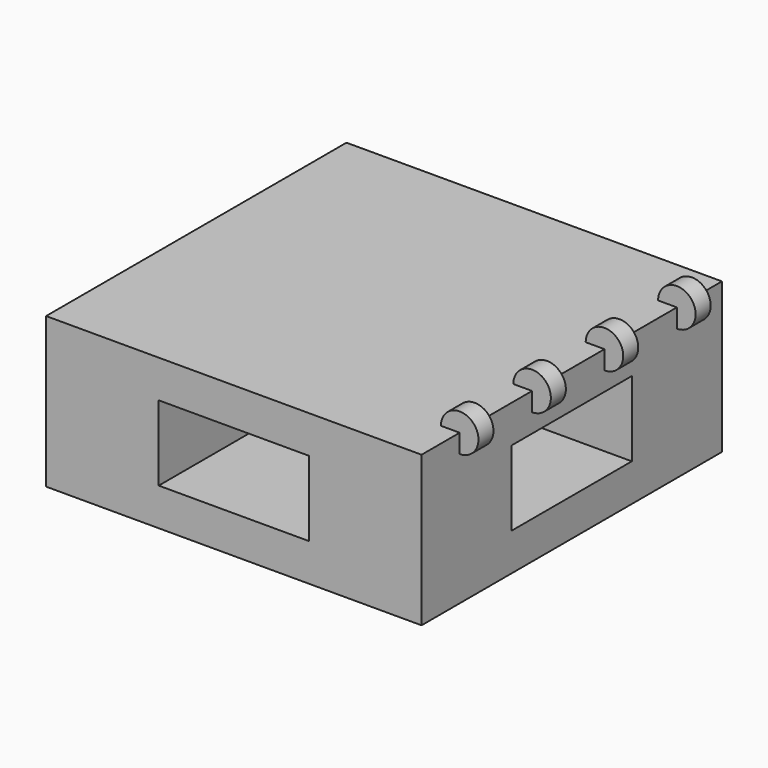
from build123d import *

# Parameters (mm, degrees)
F0_W     = 100
F0_H     = 100
F1_DEPTH = 10
F2_W     = 30
F2_H     = 30
F3_DEPTH = 20
F5_W     = 100
F5_H     = 100
F6_DEPTH = 10
F7_W     = 5
F7_H     = 5


with BuildPart() as f1:
    # F0 (on Top) → F1 (new body)
    with BuildSketch(Plane.XY):
        Rectangle(F0_W, F0_H)
    extrude(amount=F1_DEPTH)

    # F2 (on face) → F3 (join)
    with BuildSketch(Plane.XY.offset(10)):
        with Locations((-35, 35)):
            Rectangle(F2_W, F2_H)
        with Locations((35, 35)):
            Rectangle(F2_W, F2_H)
        with Locations((-35, -35)):
            Rectangle(F2_W, F2_H)
        with Locations((35, -35)):
            Rectangle(F2_W, F2_H)
    extrude(amount=F3_DEPTH)

    # F5 (on offset) → F6 (join)
    with BuildSketch(Plane.XY.offset(30)):
        Rectangle(F5_W, F5_H)
    extrude(amount=F6_DEPTH)

    # F7 (on face) → F8 (revolve)
    with BuildSketch(Plane.XY.offset(40)):
        with Locations((47.5, 37.5)):
            Rectangle(F7_W, F7_H)
        with Locations((47.5, 13.3981328524)):
            Rectangle(F7_W, F7_H)
        with Locations((47.5, -10.7037342952)):
            Rectangle(F7_W, F7_H)
        with Locations((47.5, -34.8056014428)):
            Rectangle(F7_W, F7_H)
    revolve(axis=Axis((50, 0, 40), (0, -1, 0)))


solid = f1.part
